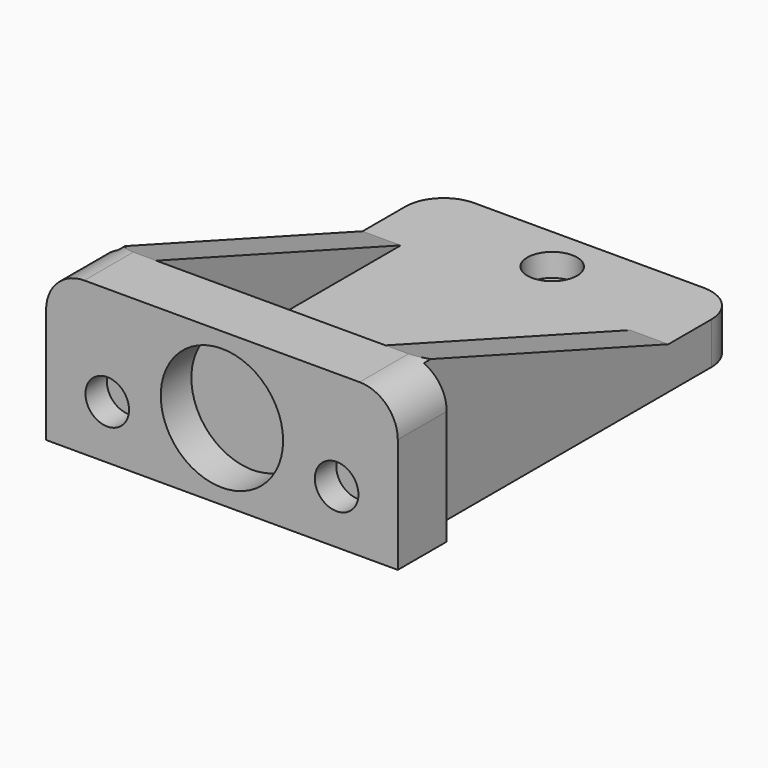
from build123d import *

# Parameters (mm, degrees)
F0_W           = 3
F0_H           = 8
F1_DEPTH       = 20
F0_W_2         = 30
F0_H_2         = 12
F0_H_3         = 40
F0_W_3         = 5
F2_DEPTH       = 5.5
F3_DEPTH       = 20
F5_DEPTH       = 43.001
F7_D           = 3.3
F7_DEPTH       = 13.5002857143
F7_CBORE_D     = 6.5
F7_CBORE_DEPTH = 3
F7_TIP         = 0.9914200214
F8_R           = 8
F9_DEPTH       = 5
F8_R_2         = 2.85
F10_DEPTH      = 3.5
F11_T1_DEPTH   = 30.5
F11_T3_DEPTH   = 33


# Not quite as in the source:
# - a fillet or chamfer that OpenCascade refuses, or shapes differently, is made with other operations: its cross-section is extruded or revolved along the edge and cut away or added


with BuildPart() as f1:
    # F0 (on Top) → F1 (new body)
    with BuildSketch(Plane.XY):
        Polygon((20, -30), (20, -22), (15, -22), (-15, -22), (-20, -22), (-20, -30), align=None)
        with Locations((-21.5, -26)):
            Rectangle(F0_W, F0_H)
        with Locations((21.5, -26)):
            Rectangle(F0_W, F0_H)
    extrude(amount=F1_DEPTH)

    # F0 (on Top) → F2 (join)
    with BuildSketch(Plane.XY):
        with Locations((0, 24)):
            Rectangle(F0_W_2, F0_H_2)
        with Locations((0, -2)):
            Rectangle(F0_W_2, F0_H_3)
        with Locations((-17.5, 24)):
            Rectangle(F0_W_3, F0_H_2)
        with Locations((-17.5, -2)):
            Rectangle(F0_W_3, F0_H_3)
        with Locations((17.5, 24)):
            Rectangle(F0_W_3, F0_H_2)
        with Locations((17.5, -2)):
            Rectangle(F0_W_3, F0_H_3)
    extrude(amount=F2_DEPTH)

    # F0 (on Top) → F3 (join)
    with BuildSketch(Plane.XY):
        with Locations((-17.5, -2)):
            Rectangle(F0_W_3, F0_H_3)
        with Locations((17.5, -2)):
            Rectangle(F0_W_3, F0_H_3)
    extrude(amount=F3_DEPTH)

    # F4 (on face) → F5 (cut, through all)
    with BuildSketch(Plane(origin=(-20, 0, 0), x_dir=(0, -1, 0), z_dir=(-1, 0, 0))):
        Polygon((-18, 20), (-18, 5.5), (22, 20), align=None)
    extrude(amount=-F5_DEPTH, mode=Mode.SUBTRACT)

    # F7
    with Locations(Plane.XY.offset(5.5)):
        with Locations((0, 24), (0, -16)):
            CounterBoreHole(F7_D / 2, F7_CBORE_D / 2, F7_CBORE_DEPTH, depth=F7_DEPTH)
            with Locations((0, 0, -(F7_DEPTH + F7_TIP / 2))):  # 118° drill point
                Cone(0, F7_D / 2, F7_TIP, mode=Mode.SUBTRACT)

    # F8 (on face) → F9 (cut)
    with BuildSketch(Plane.XZ.offset(30)):
        with Locations((0, 10)):
            Circle(F8_R)
    extrude(amount=-F9_DEPTH, mode=Mode.SUBTRACT)

    # F8 (on face) → F10 (cut)
    with BuildSketch(Plane.XZ.offset(30)):
        with Locations((-15, 7)):
            Circle(F8_R_2)
        with Locations((15, 7)):
            Circle(F8_R_2)
    extrude(amount=-F10_DEPTH, mode=Mode.SUBTRACT)

    # F11: fillet of radius 5 on 4 edges, made by hand

    # F11_s2 → F11_t1 (cut)
    with BuildSketch(Plane.XY.offset(-12.5)):
        with BuildLine():
            ThreePointArc((15, 30), (18.5355339059, 28.5355339059), (20, 25))
            Line((20, 25), (20, 30))
            Line((20, 30), (15, 30))
        make_face()
        with BuildLine():
            ThreePointArc((-20, 25), (-18.5355339059, 28.5355339059), (-15, 30))
            Line((-15, 30), (-20, 30))
            Line((-20, 30), (-20, 25))
        make_face()
    extrude(amount=F11_T1_DEPTH, mode=Mode.SUBTRACT)

    # F11_s4 → F11_t3 (cut)
    with BuildSketch(Plane.XZ.offset(9.5)):
        with BuildLine():
            ThreePointArc((-23, 15), (-21.5355339059, 18.5355339059), (-18, 20))
            Line((-18, 20), (-23, 20))
            Line((-23, 20), (-23, 15))
        make_face()
        with BuildLine():
            ThreePointArc((18, 20), (21.5355339059, 18.5355339059), (23, 15))
            Line((23, 15), (23, 20))
            Line((23, 20), (18, 20))
        make_face()
    extrude(amount=F11_T3_DEPTH, mode=Mode.SUBTRACT)


solid = f1.part
